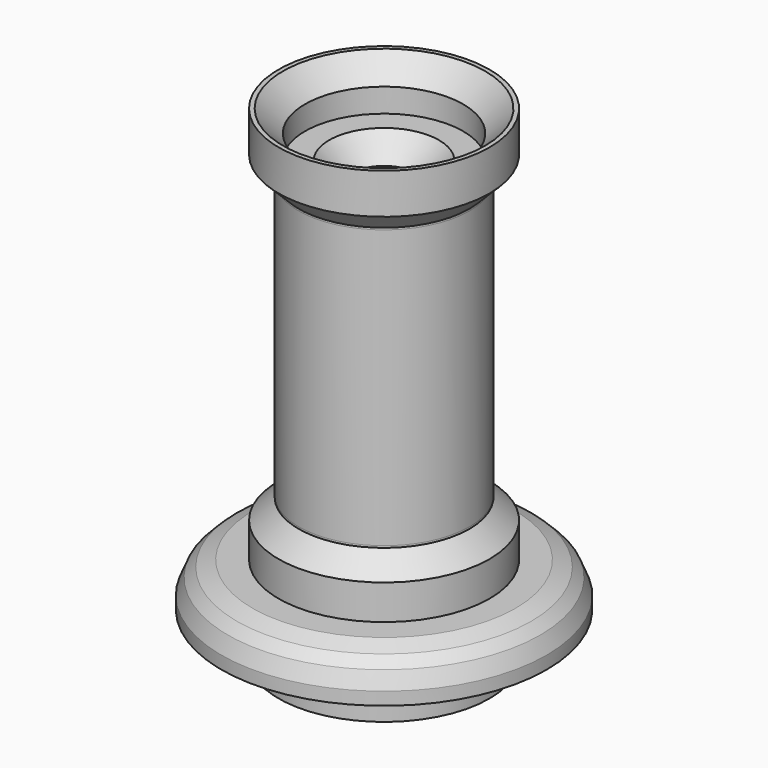
from build123d import *

# Parameters (mm, degrees)
F0_W         = 6.096
F0_H         = 5.08
F0_W_2       = 3.048
F0_H_2       = 5.2907199979
F0_W_3       = 6.604
F2_SIZE      = 2.54
F3_SIZE      = 2.54
F5_D         = 7.62
F5_DEPTH     = 25.4
F5_TIP       = 2.2892789585
F6_W         = 7.272795774
F6_H         = 32.1356244385
F8_S5_R      = 9.8747471347
F8_T6_DEPTH  = 19
F8_S11_R     = 9.8747471347
F8_T12_DEPTH = 19


# Not quite as in the source:
# - a fillet or chamfer that OpenCascade refuses, or shapes differently, is made with other operations: its cross-section is extruded or revolved along the edge and cut away or added


with BuildPart() as f1:
    # F0 (on Front) → F1 (revolve)
    with BuildSketch(Plane.XZ):
        with Locations((9.144, 2.54)):
            Rectangle(F0_W, F0_H)
        Polygon((0, 50.8), (0, 47.4797748029), (6.096, 50.8), align=None)
        with Locations((9.144, 7.62)):
            Rectangle(F0_W, F0_H)
        with Locations((10.668, 53.4453599989)):
            Rectangle(F0_W_2, F0_H_2)
        Polygon((0, 47.4797748029), (0, 0), (6.096, 0), (6.096, 5.08), (6.096, 10.16), (12.192, 10.16), (12.192, 50.8), (9.144, 50.8), (6.096, 50.8), align=None)
        with Locations((15.494, 7.62)):
            Rectangle(F0_W_3, F0_H)
    revolve(axis=Axis((0, 0, 25.4), (0, 0, 1)))

    # F2
    f2_edges = [f1.edges().sort_by_distance(p)[0] for p in [
        (-9.144, 0, 56.09072),
    ]]
    chamfer(f2_edges, length=F2_SIZE)

    # F3
    f3_edges = [f1.edges().sort_by_distance(p)[0] for p in [
        (-18.796, 0, 10.16),
    ]]
    chamfer(f3_edges, length=F3_SIZE)

    # F5
    with Locations(Plane.XY.offset(50.8)):
        with Locations((0, 0)):
            Hole(F5_D / 2, depth=F5_DEPTH)
            with Locations((0, 0, -(F5_DEPTH + F5_TIP / 2))):  # 118° drill point
                Cone(0, F5_D / 2, F5_TIP, mode=Mode.SUBTRACT)

    # F6 (on Right) → F7 (revolve, cut)
    with BuildSketch(Plane.YZ):
        with Locations((-13.5111450218, 32.7963028103)):
            Rectangle(F6_W, F6_H)
    revolve(axis=Axis((0, 0, 32.7963028103), (0, 0, -1)), mode=Mode.SUBTRACT)

    # F8: chamfer of 2.54 on 5 edges, made by hand


with BuildPart() as f8_tool2:
    # F8_s3 → F8_t4 (revolve)
    with BuildSketch(Plane.XZ):
        Polygon((9.652, 48.8641150296), (12.192, 51.4041150296), (12.192, 48.8641150296), align=None)
    revolve(axis=Axis((0, 0, 48.8641150296), (0, 0, 1)))

    # F8_s5 → F8_t6 (cut, symmetric)
    with BuildSketch(Plane.XY.offset(50.1)):
        Circle(F8_S5_R)
    extrude(amount=F8_T6_DEPTH, both=True, mode=Mode.SUBTRACT)


with BuildPart() as f1_1:
    add(f1.part)

    # F8_t1: cut F8_tool2
    add(f8_tool2.part, mode=Mode.SUBTRACT)


with BuildPart() as f8_tool8:
    # F8_s9 → F8_t10 (revolve)
    with BuildSketch(Plane.XZ):
        Polygon((12.192, 14.188490591), (9.652, 16.728490591), (12.192, 16.728490591), align=None)
    revolve(axis=Axis((0, 0, 16.728490591), (0, 0, 1)))

    # F8_s11 → F8_t12 (cut, symmetric)
    with BuildSketch(Plane.XY.offset(15.5)):
        Circle(F8_S11_R)
    extrude(amount=F8_T12_DEPTH, both=True, mode=Mode.SUBTRACT)


with BuildPart() as f1_2:
    add(f1_1.part)

    # F8_t7: cut F8_tool8
    add(f8_tool8.part, mode=Mode.SUBTRACT)

    # F8_s13 → F8_t14 (revolve, cut)
    with BuildSketch(Plane.XZ):
        Polygon((15.2038975516, 10.16), (16.9999487758, 9.4160512242), (16.256, 10.16), align=None)
    revolve(axis=Axis((0, 0, 10.16), (0, 0, 1)), mode=Mode.SUBTRACT)

    # F8_s15 → F8_t16 (revolve, cut)
    with BuildSketch(Plane.XZ):
        Polygon((18.0520512242, 8.3639487758), (18.796, 6.5678975516), (18.796, 7.62), align=None)
    revolve(axis=Axis((0, 0, 7.62), (0, 0, 1)), mode=Mode.SUBTRACT)

    # F8_s17 → F8_t18 (revolve, cut)
    with BuildSketch(Plane.XZ):
        Polygon((6.35, 50.8), (3.81, 48.26), (3.81, 50.8), align=None)
    revolve(axis=Axis((0, 0, 50.8), (0, 0, 1)), mode=Mode.SUBTRACT)


solid = f1_2.part
